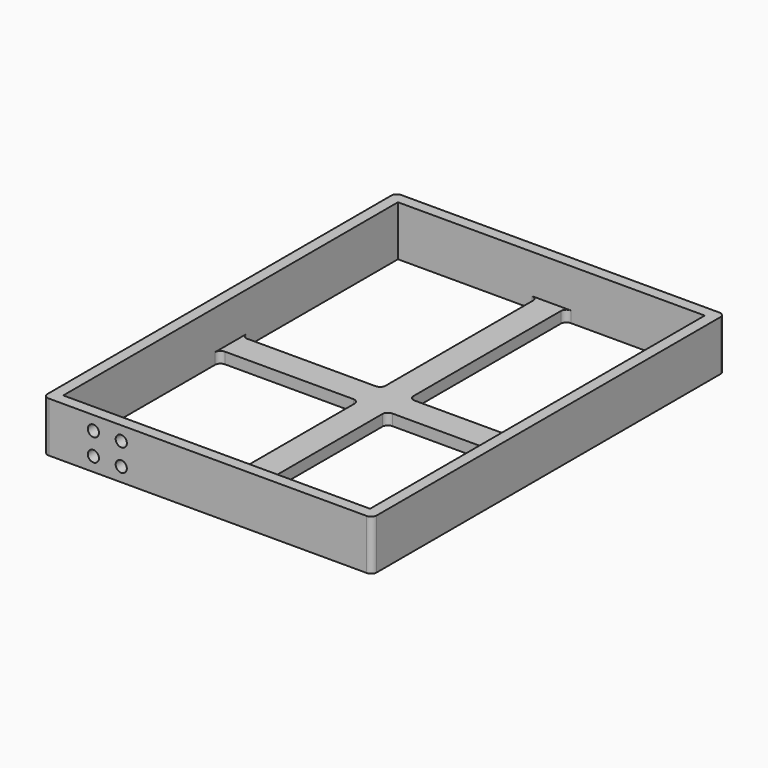
from build123d import *

# Parameters (mm, degrees)
F0_W     = 59
F0_H     = 79
F0_W_2   = 55
F0_H_2   = 75
F1_DEPTH = 9
F3_DEPTH = 2
F4_R     = 1
F5_DEPTH = 2.001
F6_R     = 1
F9_DEPTH = 11
F10_R    = 0.99999


# Not quite as in the source:
# - two fillets or chamfers of one size are made in one step
# - a fillet or chamfer is up to 0.001 mm smaller than in the source, because OpenCascade refuses the exact size


with BuildPart() as f1:
    # F0 (on Top) → F1 (new body)
    with BuildSketch(Plane.XY):
        Rectangle(F0_W, F0_H)
        Rectangle(F0_W_2, F0_H_2, mode=Mode.SUBTRACT)
    extrude(amount=F1_DEPTH)

    # F2 (on Top) → F3 (join)
    with BuildSketch(Plane.XY):
        Polygon((2.5, 38.5), (-2.5, 38.5), (-2.5, 2.5), (-28.5, 2.5), (-28.5, -2.5), (-2.5, -2.5), (-2.5, -38.5), (2.5, -38.5), (2.5, -2.5), (28.5, -2.5), (28.5, 2.5), (2.5, 2.5), align=None)
    extrude(amount=F3_DEPTH)

    # F4 (on face) → F5 (cut, through all)
    with BuildSketch(Plane(origin=(0, -37.5, 0), x_dir=(-1, 0, 0), z_dir=(0, 1, 0))):
        with Locations((20.5, 2.5)):
            Circle(F4_R)
        with Locations((20.5, 6.5)):
            Circle(F4_R)
        with Locations((15.5, 2.5)):
            Circle(F4_R)
        with Locations((15.5, 6.5)):
            Circle(F4_R)
    extrude(amount=-F5_DEPTH, mode=Mode.SUBTRACT)

    # F6
    f6_edges = [f1.edges().sort_by_distance(p)[0] for p in [
        (-29.5, -39.5, 4.5),
        (29.5, -39.5, 4.5),
        (-29.5, 39.5, 4.5),
        (29.5, 39.5, 4.5),
        (-2.5, 2.5, 1),
        (2.5, 2.5, 1),
        (2.5, -2.5, 1),
        (-2.5, -2.5, 1),
        (2.5, -37.5, 1),
        (-2.5, -37.5, 1),
        (-27.5, -2.5, 1),
        (-27.5, 2.5, 1),
        (27.5, -2.5, 1),
        (27.5, 2.5, 1),
        (2.5, 37.5, 1),
        (-2.5, 37.5, 1),
    ]]
    fillet(f6_edges, radius=F6_R)

    # F8 (on offset) → F9 (join)
    with BuildSketch(Plane.YZ.offset(-23.5)):
        with BuildLine():
            ThreePointArc((-37.5, 3.5), (-36.5, 4.5), (-37.5, 5.5))
            Line((-37.5, 5.5), (-37.5, 3.5))
        make_face()
    extrude(amount=F9_DEPTH)

    # F10 (radius 1 in the source; OpenCascade refuses exactly that, so slightly less here)
    f10_edges = [f1.edges().sort_by_distance(p)[0] for p in [
        (-23.5, -36.5, 4.5),
        (-12.5, -36.5, 4.5),
    ]]
    fillet(f10_edges, radius=F10_R)


solid = f1.part
